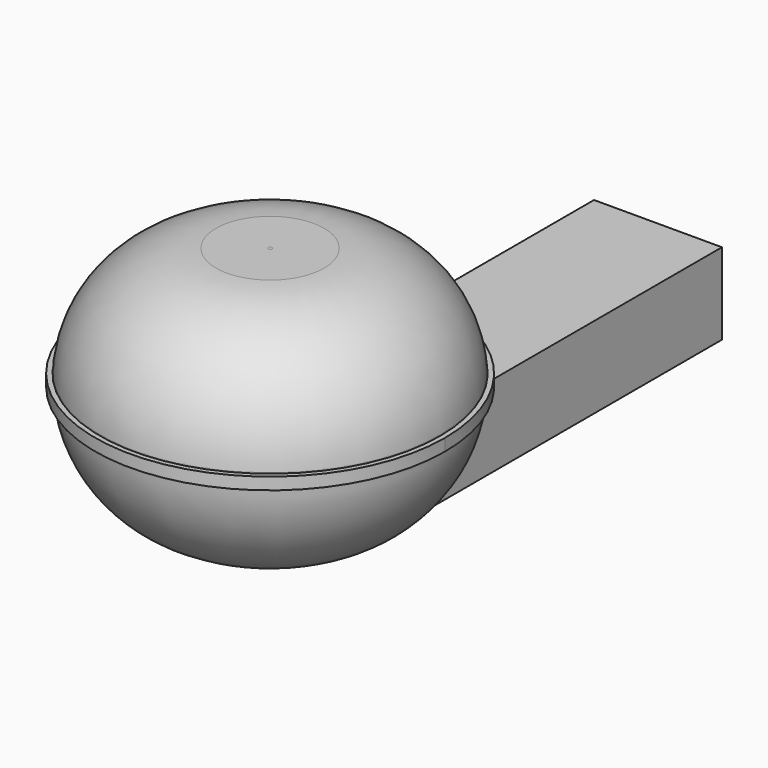
from build123d import *

# Parameters (mm, degrees)
F0_W     = 69.7972998023
F0_H     = 122.7901950479
F1_DEPTH = 55.8849815279
F3_W     = 53.2010421157
F3_H     = 168.4204190969
F4_DEPTH = 33.8678937405
F6_DEPTH = 5.0218440592
F7_R     = 70.6929415692
F8_DEPTH = 50.8
F9_DEPTH = 101.6
F11_R    = 48.2263241047


# Not quite as in the source:
# - a fillet or chamfer that OpenCascade refuses, or shapes differently, is made with other operations: its cross-section is extruded or revolved along the edge and cut away or added


with BuildPart() as f1:
    # F0 (on Top) → F1 (new body)
    with BuildSketch(Plane.XY):
        with Locations((49.6131367981, 5.3991861641)):
            Rectangle(F0_W, F0_H)
    extrude(amount=F1_DEPTH)


with BuildPart() as f4:
    # F3 (on Top) → F4 (new body)
    with BuildSketch(Plane.XY):
        with Locations((37.3318605125, -6.2110945582)):
            Rectangle(F3_W, F3_H)
    extrude(amount=F4_DEPTH)

    # F5 (on face) → F6 (join)
    with BuildSketch(Plane.XY.offset(33.8678937405)):
        with BuildLine():
            ThreePointArc((10.7313394546, -17.6587030794), (-40.7195891486, -141.8722327099), (83.493940482, -90.4213041067))
            ThreePointArc((83.493940482, -90.4213041067), (78.4271381056, -63.7440674942), (63.9323815703, -40.7821539723))
            Line((63.9323815703, -40.7821539723), (63.9323815703, -90.4213041067))
            Line((63.9323815703, -90.4213041067), (10.7313394547, -90.4213041067))
            Line((10.7313394547, -90.4213041067), (10.7313394547, -17.6587030794))
        make_face()
        with BuildLine():
            Line((63.9323815703, -90.4213041067), (63.9323815703, -40.7821539723))
            ThreePointArc((63.9323815703, -40.7821539723), (39.7358428265, -23.6894909108), (10.7313394546, -17.6587030794))
            Line((10.7313394547, -17.6587030794), (10.7313394547, -90.4213041067))
            Line((10.7313394547, -90.4213041067), (63.9323815703, -90.4213041067))
        make_face()
    extrude(amount=F6_DEPTH)

    # F7 (on face) → F8 (join)
    with BuildSketch(Plane.XY.offset(33.8678937405)):
        with Locations((10.7313394547, -90.4213041067)):
            Circle(F7_R)
    extrude(amount=F8_DEPTH)


with BuildPart() as f9:
    # F9 (new): a face of the model
    f9_faces = [f4.part.faces().sort_by_distance(p)[0] for p in [
        (10.7313394547, -90.4213041067, 84.6678937405),
    ]]
    extrude(f9_faces, amount=-F9_DEPTH)

    # F11
    f11_edges = [f9.edges().sort_by_distance(p)[0] for p in [
        (-59.961602, -90.421304, 84.667894),
    ]]
    fillet(f11_edges, radius=F11_R)

    # F12: fillet of radius 53.7061455259 on 1 edges, made by hand

    # F12_s1 → F12_t2 (revolve, cut)
    with BuildSketch(Plane.XZ.offset(90.4213041067)):
        with BuildLine():
            ThreePointArc((81.4242810238, 36.4415696358), (65.5774160343, -1.3193048347), (27.7191645897, -16.9321062595))
            Line((27.7191645897, -16.9321062595), (27.7191645897, -18.00622917))
            Line((27.7191645897, -18.00622917), (81.4242810238, -18.00622917))
            Line((81.4242810238, -18.00622917), (82.4984039343, -16.9321062595))
            Line((82.4984039343, -16.9321062595), (82.4983833525, 36.4349202432))
            Line((82.4983833525, 36.4349202432), (81.4242810238, 36.4415696358))
        make_face()
    revolve(axis=Axis((10.7313394547, -90.4213041067, -16.9321062595), (0, 0, 1)), mode=Mode.SUBTRACT)


with BuildPart() as f4_1:
    add(f4.part)

    # F10: fillet of radius 76.2 on 1 edges, made by hand

    # F10_s1 → F10_t2 (revolve, cut)
    with BuildSketch(Plane.XZ.offset(90.4213041067)):
        with BuildLine():
            ThreePointArc((81.4242810238, 38.8897377998), (53.3234697948, 72.2040079824), (11.5604749148, 84.6678937405))
            Line((11.5604749148, 84.6678937405), (81.4242810238, 84.6678937405))
            Line((81.4242810238, 84.6678937405), (81.4242810238, 38.8897377998))
        make_face()
    revolve(axis=Axis((10.7313394547, -90.4213041067, 84.6678937405), (0, 0, 1)), mode=Mode.SUBTRACT)


solid = Compound([f9.part, f4_1.part])
